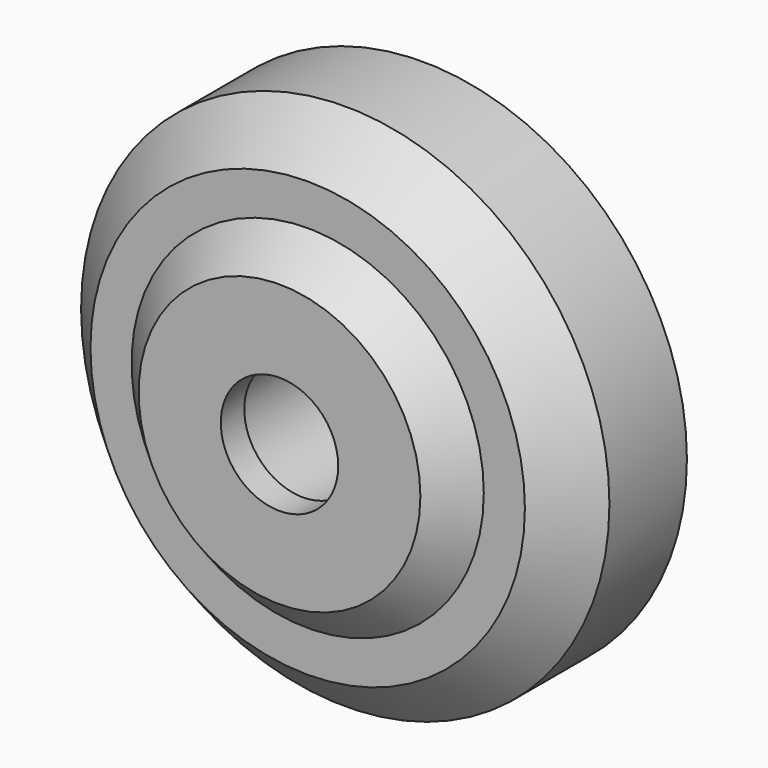
from build123d import *

# Parameters (mm, degrees)
F0_R      = 45
F1_DEPTH  = 25.5
F2_R      = 58
F3_DEPTH  = 1
F4_SIZE   = 8
F5_R      = 30
F6_DEPTH  = 6
F7_SIZE   = 5.99999
F9_R      = 11
F10_DEPTH = 25
F11_R     = 11
F11_R_2   = 10
F12_DEPTH = 5


# Not quite as in the source:
# - a fillet or chamfer is up to 0.001 mm smaller than in the source, because OpenCascade refuses the exact size


with BuildPart() as f1:
    # F0 (on Front) → F1 (new body)
    with BuildSketch(Plane.XZ):
        Circle(F0_R)
    extrude(amount=F1_DEPTH)

    # F2 (on face) → F3 (cut)
    with BuildSketch(Plane(origin=(0, 0, 0), x_dir=(-1, 0, 0), z_dir=(0, 1, 0))):
        Circle(F2_R)
    extrude(amount=-F3_DEPTH, mode=Mode.SUBTRACT)

    # F4
    f4_edges = [f1.edges().sort_by_distance(p)[0] for p in [
        (-45, -25.5, 0),
    ]]
    chamfer(f4_edges, length=F4_SIZE)

    # F5 (on face) → F6 (join)
    with BuildSketch(Plane.XZ.offset(25.5)):
        Circle(F5_R)
    extrude(amount=F6_DEPTH)

    # F7 (size 6 in the source; OpenCascade refuses exactly that, so slightly less here)
    f7_edges = [f1.edges().sort_by_distance(p)[0] for p in [
        (-30, -31.5, 0),
    ]]
    chamfer(f7_edges, length=F7_SIZE)

    # F9 (on face) → F10 (cut)
    with BuildSketch(Plane.XZ.offset(31.5)):
        Circle(F9_R)
    extrude(amount=-F10_DEPTH, mode=Mode.SUBTRACT)

    # F11 (on face) → F12 (join)
    with BuildSketch(Plane.XZ.offset(31.5)):
        Circle(F11_R)
        Circle(F11_R_2, mode=Mode.SUBTRACT)
    extrude(amount=-F12_DEPTH)


solid = f1.part
